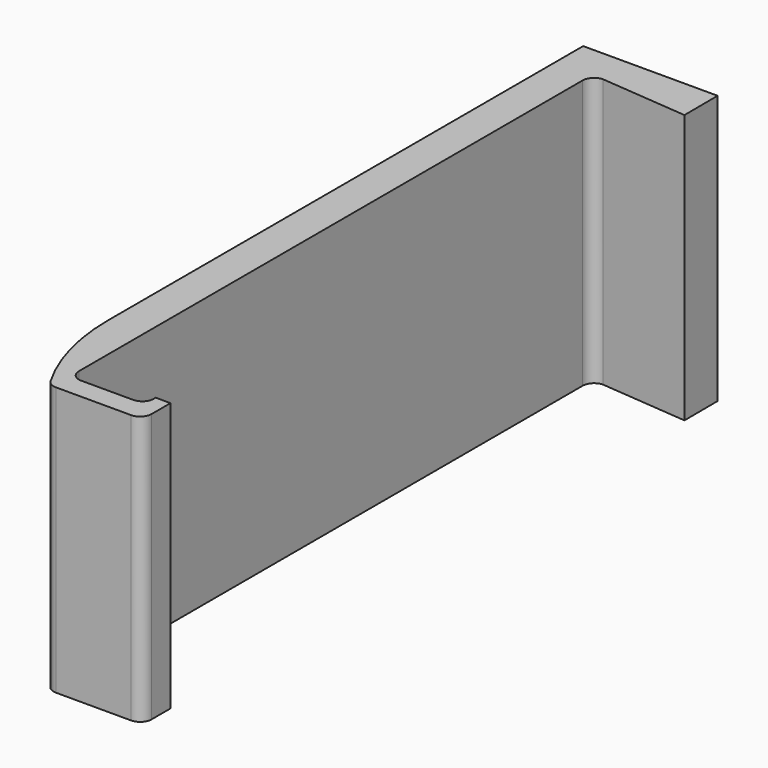
from build123d import *

# Parameters (mm, degrees)
F1_DEPTH = 30


# Not quite as in the source:
# - a feature names something its author has since deleted; it is built from what else it names


with BuildPart() as f1:
    # F0 (on Top) → F1 (new body)
    with BuildSketch(Plane.XY):
        with BuildLine():
            Line((15.0259537622, 74.3470937014), (15, 79))
            Line((15, 79), (0, 79))
            Line((0, 79), (0, 12.7))
            ThreePointArc((0, 12.7), (0.8280772268, 6.4500404007), (3.2551662494, 0.6313682358))
            ThreePointArc((3.2551662494, 0.6313682358), (3.719732188, 0.1690998364), (4.352913702, 0))
            Line((4.352913702, 0), (12.7432, 0))
            ThreePointArc((12.7432, 0), (13.6412256121, 0.3719743879), (14.0132, 1.27))
            Line((14.0132, 1.27), (14.0132, 3.9116))
            Line((14.0132, 3.9116), (12.3622, 3.9116))
            Line((12.3622, 3.9116), (12.3622, 3.6322))
            ThreePointArc((12.3622, 3.6322), (11.9902256121, 2.7341743879), (11.0922, 2.3622))
            Line((11.0922, 2.3622), (5.2832, 2.3622))
            ThreePointArc((5.2832, 2.3622), (4.3851743879, 2.7341743879), (4.0132, 3.6322))
            Line((4.0132, 3.6322), (4.0132, 73.92))
            ThreePointArc((4.0132, 73.92), (4.3851743879, 74.8180256121), (5.2832, 75.19))
            Line((5.2832, 75.19), (15.0259537622, 74.3470937014))
        make_face()
    extrude(amount=F1_DEPTH)


solid = f1.part
